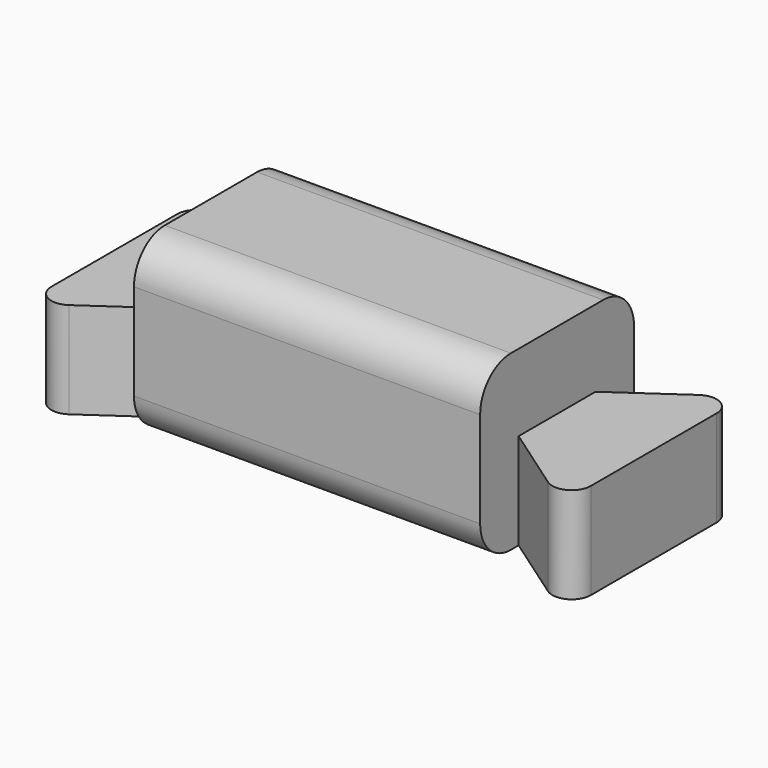
from build123d import *

# Parameters (mm, degrees)
F1_DEPTH = 9
F2_R     = 2
F3_DEPTH = 5
F4_R     = 1


with BuildPart() as f1:
    # F0 (on Top) → F1 (new body)
    with BuildSketch(Plane.XY):
        Polygon((9, 5), (0, 5), (-9, 5), (-9, 2.5), (-9, -2.5), (-9, -5), (0, -5), (9, -5), (9, -2.5), (9, 0), (9, 2.5), align=None)
    extrude(amount=F1_DEPTH)

    # F2
    f2_edges = [f1.edges().sort_by_distance(p)[0] for p in [
        (0, -5, 9),
        (0, 5, 9),
        (0, 5, 0),
        (0, -5, 0),
    ]]
    fillet(f2_edges, radius=F2_R)

    # F0 (on Top) → F3 (join)
    with BuildSketch(Plane.XY):
        Polygon((14.0249378106, 6), (9, 2.5), (9, 0), (14.0249378106, 0), align=None)
        Polygon((14.0249378106, 0), (9, 0), (9, -2.5), (14.0249378106, -6), align=None)
        Polygon((-9, -2.5), (-9, 2.5), (-14.0249378106, 6), (-14.0249378106, -6), align=None)
    extrude(amount=F3_DEPTH)

    # F4
    f4_edges = [f1.edges().sort_by_distance(p)[0] for p in [
        (-14.024938, 6, 2.5),
        (-14.024938, -6, 2.5),
        (14.024938, -6, 2.5),
        (14.024938, 6, 2.5),
    ]]
    fillet(f4_edges, radius=F4_R)


solid = f1.part
